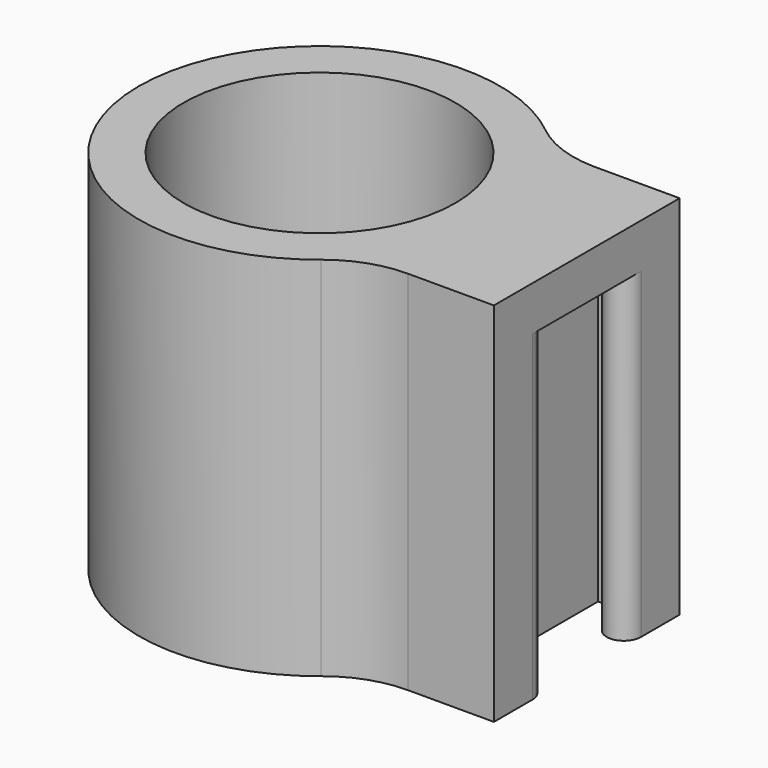
from build123d import *

# Parameters (mm, degrees)
F0_R     = 9.652
F1_DEPTH = 22.86
F2_R     = 9.652
F3_DEPTH = 3.175
F4_R     = 9.652
F5_DEPTH = 3.175


with BuildPart() as f1:
    # F0 (on Top) → F1 (new body)
    with BuildSketch(Plane.XY):
        with BuildLine():
            Line((14.4724995292, -6.4216016291), (14.4724995292, 6.2783983709))
            Line((14.4724995292, 6.2783983709), (14.4724995292, 6.6347159585))
            Line((14.4724995292, 6.6347159585), (14.5994995292, 6.6347159585))
            Line((14.5994995292, 6.6347159585), (16.1869995292, 6.6347159585))
            Line((16.1869995292, 6.6347159585), (16.5567258399, 6.6347159585))
            Line((16.5567258399, 6.6347159585), (16.5567258399, 4.7932159585))
            ThreePointArc((16.5567258399, 4.7932159585), (17.7744995292, 3.5754422692), (18.9922732184, 4.7932159585))
            Line((18.9922732184, 4.7932159585), (18.9922732184, 6.6347159585))
            Line((18.9922732184, 6.6347159585), (18.9922732184, 8.2222159585))
            Line((18.9922732184, 8.2222159585), (14.4724995292, 8.2222159585))
            Line((14.4724995292, 8.2222159585), (12.8849995292, 8.2222159585))
            ThreePointArc((12.8849995292, 8.2222159585), (10.3328098948, 8.6905993264), (8.0737784074, 9.9672479265))
            ThreePointArc((8.0737784074, 9.9672479265), (-12.827, 0), (8.0737784074, -9.9672479265))
            ThreePointArc((8.0737784074, -9.9672479265), (10.3329433344, -8.7017229937), (12.8849995292, -8.2631016291))
            Line((12.8849995292, -8.2631016291), (14.4724995292, -8.2631016291))
            Line((14.4724995292, -8.2631016291), (18.9922732184, -8.2631016291))
            Line((18.9922732184, -8.2631016291), (18.9922732184, -6.6756016291))
            Line((18.9922732184, -6.6756016291), (18.9922732184, -4.8341016291))
            ThreePointArc((18.9922732184, -4.8341016291), (17.7744995292, -3.6163279398), (16.5567258399, -4.8341016291))
            Line((16.5567258399, -4.8341016291), (16.5567258399, -6.6756016291))
            Line((16.5567258399, -6.6756016291), (16.1869995292, -6.6756016291))
            Line((16.1869995292, -6.6756016291), (14.4724995292, -6.6756016291))
            Line((14.4724995292, -6.6756016291), (14.4724995292, -6.4216016291))
        make_face()
        Circle(F0_R, mode=Mode.SUBTRACT)
    extrude(amount=F1_DEPTH)

    # F2 (on face) → F3 (join)
    with BuildSketch(Plane.XY.offset(22.86)):
        with BuildLine():
            ThreePointArc((12.8849995292, 8.2222159585), (10.3328098948, 8.6905993264), (8.0737784074, 9.9672479265))
            ThreePointArc((8.0737784074, 9.9672479265), (-12.827, 0), (8.0737784074, -9.9672479265))
            ThreePointArc((8.0737784074, -9.9672479265), (10.3329433344, -8.7017229937), (12.8849995292, -8.2631016291))
            Line((12.8849995292, -8.2631016291), (18.9922732184, -8.2631016291))
            Line((18.9922732184, -8.2631016291), (18.9922732184, -4.8341016291))
            ThreePointArc((18.9922732184, -4.8341016291), (17.7744995292, -3.6163279398), (16.5567258399, -4.8341016291))
            Line((16.5567258399, -4.8341016291), (16.5567258399, -6.6756016291))
            Line((16.5567258399, -6.6756016291), (14.4724995292, -6.6756016291))
            Line((14.4724995292, -6.6756016291), (14.4724995292, 6.6347159585))
            Line((14.4724995292, 6.6347159585), (16.5567258399, 6.6347159585))
            Line((16.5567258399, 6.6347159585), (16.5567258399, 4.7932159585))
            ThreePointArc((16.5567258399, 4.7932159585), (17.7744995292, 3.5754422692), (18.9922732184, 4.7932159585))
            Line((18.9922732184, 4.7932159585), (18.9922732184, 8.2222159585))
            Line((18.9922732184, 8.2222159585), (12.8849995292, 8.2222159585))
        make_face()
        Circle(F2_R, mode=Mode.SUBTRACT)
        with BuildLine():
            Line((18.9922732184, -4.8341016291), (18.9922732184, 4.7932159585))
            ThreePointArc((18.9922732184, 4.7932159585), (17.7744995292, 3.5754422692), (16.5567258399, 4.7932159585))
            Line((16.5567258399, 4.7932159585), (16.5567258399, 6.6347159585))
            Line((16.5567258399, 6.6347159585), (14.4724995292, 6.6347159585))
            Line((14.4724995292, 6.6347159585), (14.4724995292, -6.6756016291))
            Line((14.4724995292, -6.6756016291), (16.5567258399, -6.6756016291))
            Line((16.5567258399, -6.6756016291), (16.5567258399, -4.8341016291))
            ThreePointArc((16.5567258399, -4.8341016291), (17.7744995292, -3.6163279398), (18.9922732184, -4.8341016291))
        make_face()
    extrude(amount=F3_DEPTH)

    # F4 (on face) → F5 (join)
    with BuildSketch(Plane(origin=(0, 0, 0), x_dir=(1, 0, 0), z_dir=(0, 0, -1))):
        with BuildLine():
            Line((18.9922732184, 8.2631016291), (12.8849995292, 8.2631016291))
            ThreePointArc((12.8849995292, 8.2631016291), (10.3329433344, 8.7017229937), (8.0737784074, 9.9672479265))
            ThreePointArc((8.0737784074, 9.9672479265), (-12.827, 0), (8.0737784074, -9.9672479265))
            ThreePointArc((8.0737784074, -9.9672479265), (10.3328098948, -8.6905993264), (12.8849995292, -8.2222159585))
            Line((12.8849995292, -8.2222159585), (18.9922732184, -8.2222159585))
            Line((18.9922732184, -8.2222159585), (18.9922732184, -4.7932159585))
            ThreePointArc((18.9922732184, -4.7932159585), (17.7744995292, -3.5754422692), (16.5567258399, -4.7932159585))
            Line((16.5567258399, -4.7932159585), (16.5567258399, -6.6347159585))
            Line((16.5567258399, -6.6347159585), (14.4724995292, -6.6347159585))
            Line((14.4724995292, -6.6347159585), (14.4724995292, 6.6756016291))
            Line((14.4724995292, 6.6756016291), (16.5567258399, 6.6756016291))
            Line((16.5567258399, 6.6756016291), (16.5567258399, 4.8341016291))
            ThreePointArc((16.5567258399, 4.8341016291), (17.7744995292, 3.6163279398), (18.9922732184, 4.8341016291))
            Line((18.9922732184, 4.8341016291), (18.9922732184, 8.2631016291))
        make_face()
        Circle(F4_R, mode=Mode.SUBTRACT)
        Circle(F4_R)
    extrude(amount=-F5_DEPTH)


solid = f1.part
